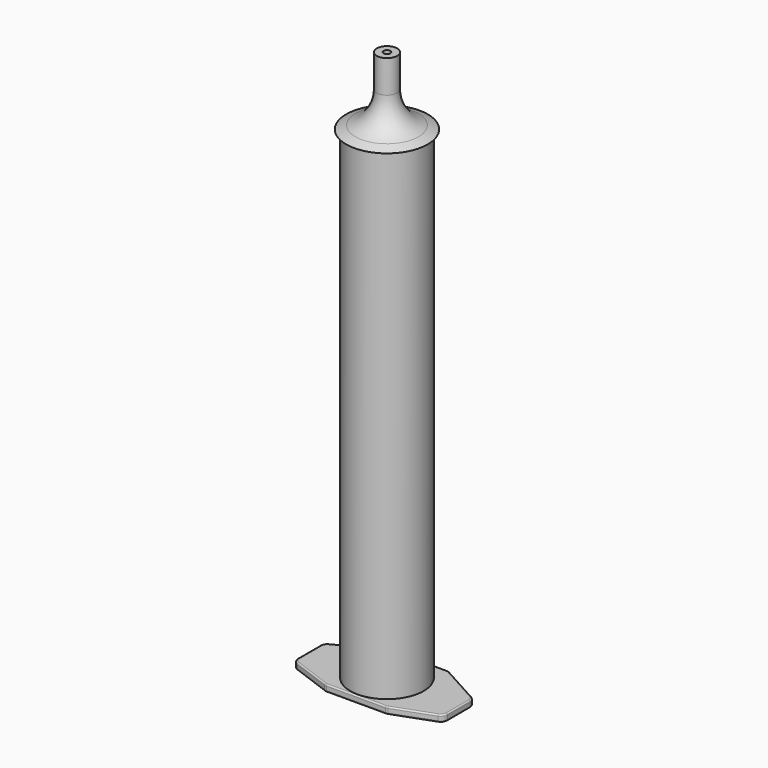
from build123d import *

# Parameters (mm, degrees)
F0_R          = 5.4
F0_R_2        = 5
F1_DEPTH      = 62
F1_DEPTH_BACK = 9
F5_R          = 5
F6_DEPTH      = 1
F7_R          = 1
F8_R          = 0.2
F9_R          = 0.2


# Not quite as in the source:
# - a feature names something its author has since deleted; it is built from what else it names


with BuildPart() as f1:
    # F0 (on Top) → F1 (new body, two sides)
    with BuildSketch(Plane.XY) as f1_sk:
        Circle(F0_R)
        Circle(F0_R_2, mode=Mode.SUBTRACT)
    extrude(amount=F1_DEPTH)
    extrude(f1_sk.sketch, amount=-F1_DEPTH_BACK)

    # F2 (on Front) → F3 (revolve)
    with BuildSketch(Plane.XZ):
        with BuildLine():
            Line((6, 62), (4.6430466171, 62.5427813535))
            ThreePointArc((4.6430466171, 62.5427813535), (2.3596638473, 64.3820207615), (1.5, 67.1851648075))
            Line((1.5, 67.1851648075), (1.5, 72))
            Line((1.5, 72), (0.5, 72))
            Line((0.5, 72), (0.5, 63.8000000012))
            Line((0.5, 63.8000000012), (5, 62))
            Line((5, 62), (6, 62))
        make_face()
    revolve(axis=Axis((0, 0, 62.4439572394), (0, 0, 1)))

    # F5 (on offset) → F6 (join)
    with BuildSketch(Plane(origin=(0, 0, -9), x_dir=(1, 0, 0), z_dir=(0, 0, -1))):
        Polygon((11, 3.3135847191), (4.4980677776, 5.7), (-4.4980677776, 5.7), (-11, 3.3135847191), (-11, -2.1135847191), (-4.4980677776, -5.7), (4.4980677776, -5.7), (11, -2.1135847191), align=None)
        Circle(F5_R, mode=Mode.SUBTRACT)
    extrude(amount=F6_DEPTH)

    # F7
    f7_edges = [f1.edges().sort_by_distance(p)[0] for p in [
        (11, 2.113585, -9.5),
        (11, -3.313585, -9.5),
        (4.498068, 5.7, -9.5),
        (4.498068, -5.7, -9.5),
        (-4.498068, 5.7, -9.5),
        (-4.498068, -5.7, -9.5),
        (-11, 2.113585, -9.5),
        (-11, -3.313585, -9.5),
    ]]
    fillet(f7_edges, radius=F7_R)

    # F8
    f8_edges = [f1.edges().sort_by_distance(p)[0] for p in [
        (-7.504731, -4.596459, -10),
        (-4.495326, -5.684572, -10),
        (0, -5.7, -10),
        (-11, -0.546125, -10),
        (-10.819926, -3.187857, -10),
        (-10.861101, 2.031572, -10),
        (-7.603269, 3.987195, -10),
        (-4.489932, 5.668408, -10),
        (0, 5.7, -10),
        (4.489932, 5.668408, -10),
        (7.603269, 3.987195, -10),
        (7.504731, -4.596459, -10),
        (4.495326, -5.684572, -10),
        (10.819926, -3.187857, -10),
        (11, -0.546125, -10),
        (10.861101, 2.031572, -10),
    ]]
    fillet(f8_edges, radius=F8_R)

    # F9
    f9_edges = [f1.edges().sort_by_distance(p)[0] for p in [
        (10.819926, -3.187857, -9),
        (11, -0.546125, -9),
        (10.861101, 2.031572, -9),
        (7.603269, 3.987195, -9),
        (4.489932, 5.668408, -9),
        (0, 5.7, -9),
        (-4.489932, 5.668408, -9),
        (-10.861101, 2.031572, -9),
        (-7.603269, 3.987195, -9),
        (7.504731, -4.596459, -9),
        (0, -5.7, -9),
        (-11, -0.546125, -9),
        (-10.819926, -3.187857, -9),
        (-4.495326, -5.684572, -9),
        (4.495326, -5.684572, -9),
        (-7.504731, -4.596459, -9),
    ]]
    fillet(f9_edges, radius=F9_R)


solid = f1.part
